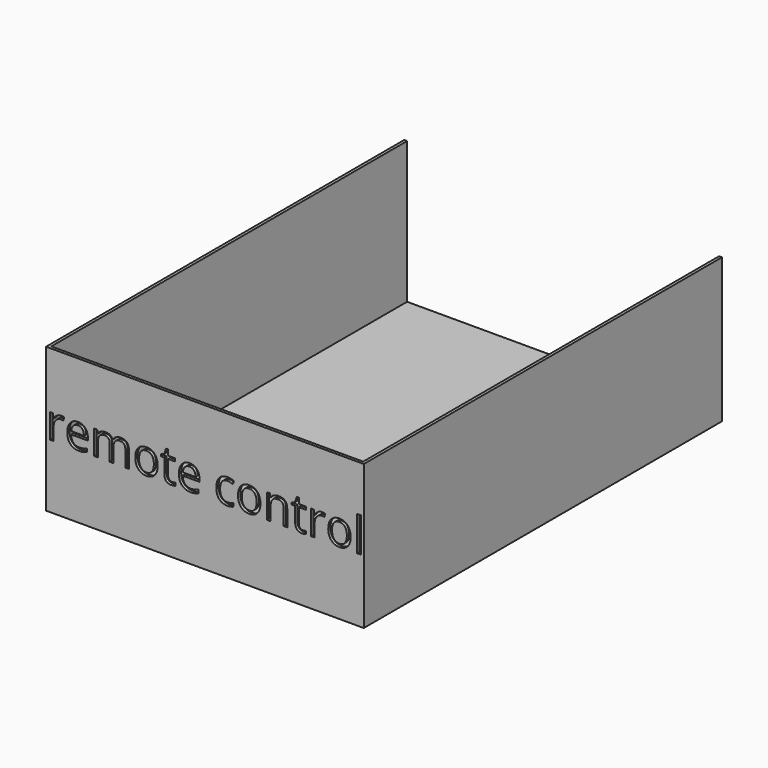
from build123d import *

# Parameters (mm, degrees)
F0_W         = 110
F0_H         = 180
F1_DEPTH     = 50
F2_T         = -1
F3_TEXT_SIZE = 15.7851072894
F4_DEPTH     = 25
F5_DEPTH     = 25


# Not quite as in the source:
# - Text() gives the source's letters only with a copy of the font that has no kerning and outlines rounded to 1/6400 em; it was checked with that copy


with BuildPart() as f1:
    # F0 (on Top) → F1 (new body)
    with BuildSketch(Plane.XY):
        Rectangle(F0_W, F0_H)
    extrude(amount=F1_DEPTH)

    # F2
    f2_openings = [f1.faces().sort_by_distance(p)[0] for p in [
        (0, 0, 50),
    ]]
    offset(amount=F2_T, openings=f2_openings)

    # F3 (on face) → F4 (cut)
    with BuildSketch(Plane.XZ.offset(90)):
        with Locations((-55, 22.0606772674)):
            Text('remote control', F3_TEXT_SIZE, font='Open Sans', text_align=(TextAlign.LEFT, TextAlign.BOTTOM))
    extrude(amount=-F4_DEPTH, mode=Mode.SUBTRACT)

    # F5 (cut): a face of the model
    f5_faces = [f1.faces().sort_by_distance(p)[0] for p in [
        (0, 90, 25),
    ]]
    extrude(f5_faces, amount=-F5_DEPTH, mode=Mode.SUBTRACT)


solid = f1.part
